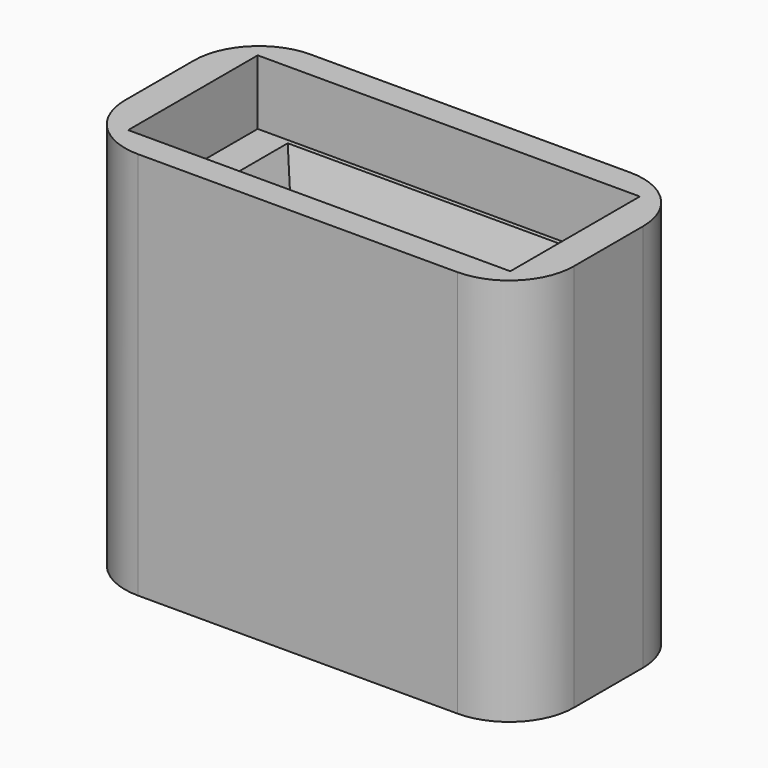
from build123d import *

# Parameters (mm, degrees)
F0_W           = 20.8
F0_H           = 10
F0_W_2         = 17.7
F0_H_2         = 7.5
F1_DEPTH       = 15
F2_DEPTH       = 3
F3_R           = 3
F4_W           = 17.7
F4_H           = 7.5
F4_W_2         = 12.6
F4_H_2         = 5.1
F5_DEPTH       = 12
F6_SIZE2       = 3
F6_SIZE        = 1
F7_TEXT_SIZE   = 8.3333333333
F7_TEXT_SIZE_2 = 5.5555555556
F8_DEPTH       = 2


# Not quite as in the source:
# - Text() gives the source's letters only with a copy of the font that has no kerning and outlines rounded to 1/6400 em; it was checked with that copy


with BuildPart() as f1:
    # F0 (on Top) → F1 (new body)
    with BuildSketch(Plane.XY):
        Rectangle(F0_W, F0_H)
        Rectangle(F0_W_2, F0_H_2, mode=Mode.SUBTRACT)
    extrude(amount=F1_DEPTH)

    # F0 (on Top) → F2 (join)
    with BuildSketch(Plane.XY):
        Rectangle(F0_W, F0_H)
        Rectangle(F0_W_2, F0_H_2, mode=Mode.SUBTRACT)
        Rectangle(F0_W_2, F0_H_2)
    extrude(amount=-F2_DEPTH)

    # F3
    f3_edges = [f1.edges().sort_by_distance(p)[0] for p in [
        (-10.4, -5, 6),
        (-10.4, 5, 6),
        (10.4, 5, 6),
        (10.4, -5, 6),
    ]]
    fillet(f3_edges, radius=F3_R)

    # F4 (on face) → F5 (join)
    with BuildSketch(Plane.XY):
        Rectangle(F4_W, F4_H)
        Rectangle(F4_W_2, F4_H_2, mode=Mode.SUBTRACT)
    extrude(amount=F5_DEPTH)

    # F6
    f6_edges = [f1.edges().sort_by_distance(p)[0] for p in [
        (0, 2.55, 12),
        (-6.3, 0, 12),
        (0, -2.55, 12),
        (6.3, 0, 12),
    ]]
    f6_side = f1.faces().sort_by_distance((8.657766, 0, 12))[0]
    chamfer(f6_edges, length=F6_SIZE, length2=F6_SIZE2, reference=f6_side)

    # F7 (on face) → F8 (cut)
    with BuildSketch(Plane(origin=(0, 0, -3), x_dir=(1, 0, 0), z_dir=(0, 0, -1))):
        with Locations((-8.8059895833, -3)):
            Text('32', F7_TEXT_SIZE, font='Open Sans', font_style=FontStyle.BOLD, text_align=(TextAlign.LEFT, TextAlign.BOTTOM))
        with Locations((0.9830729167, -3)):
            Text('GB', F7_TEXT_SIZE_2, font='Open Sans', font_style=FontStyle.BOLD, text_align=(TextAlign.LEFT, TextAlign.BOTTOM))
    extrude(amount=-F8_DEPTH, mode=Mode.SUBTRACT)


solid = f1.part
